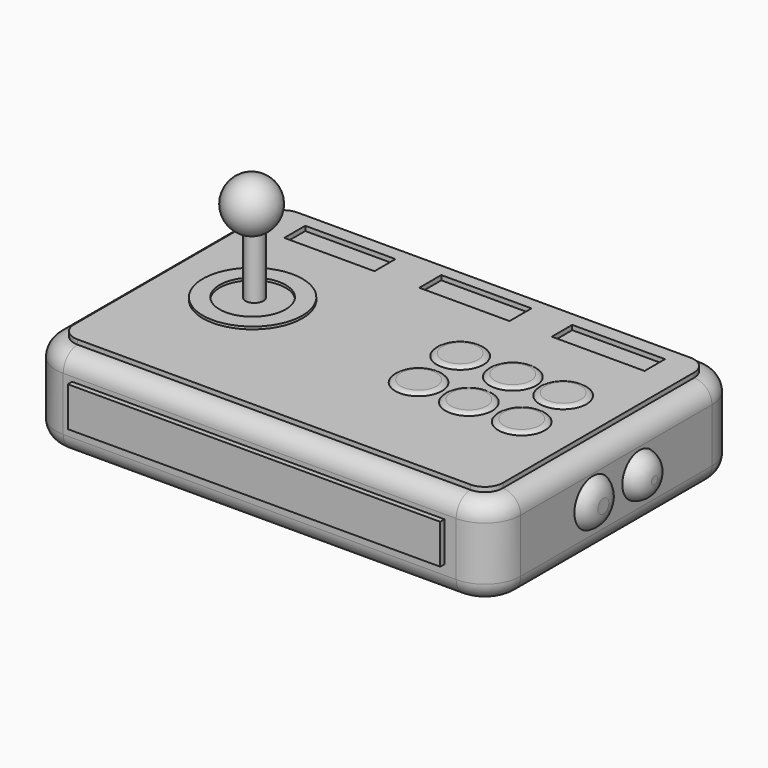
from build123d import *

# Parameters (mm, degrees)
F0_W      = 129.659101367
F0_H      = 86.704544723
F1_DEPTH  = 25
F2_R      = 10
F3_R      = 5
F4_R      = 7
F5_DEPTH  = 2
F4_R_2    = 13.8932950385
F4_R_3    = 9.2347369707
F6_R      = 1.99999
F6_2_R    = 1.99999
F6_3_R    = 1.99999
F6_4_R    = 1.99999
F6_5_R    = 1.99999
F6_6_R    = 1.99999
F7_R      = 2.4900088952
F8_DEPTH  = 18.6
F11_R     = 6.4600643812
F12_DEPTH = 2.9
F14_R     = 5.9996954232
F15_DEPTH = 4.2
F17_W     = 25.178572163
F17_H     = 7.3214266449
F17_H_2   = 7.6785702258
F17_W_2   = 25.8928574622
F17_H_3   = 7.1428548545
F18_DEPTH = 1.3
F19_W     = 22.39266783
F19_H     = 8.6377086118
F19_W_2   = 7.3178783059
F19_H_2   = 7.7066114172
F19_W_3   = 6.5572820604
F19_H_3   = 3.4711612388
F20_DEPTH = 0.7
F21_W     = 103.9311476052
F21_H     = 11.0396803357
F22_DEPTH = 1.5


# Not quite as in the source:
# - a fillet or chamfer that OpenCascade refuses, or shapes differently, is made with other operations: its cross-section is extruded or revolved along the edge and cut away or added
# - a fillet or chamfer is up to 0.001 mm smaller than in the source, because OpenCascade refuses the exact size


with BuildPart() as f1:
    # F0 (on Top) → F1 (new body)
    with BuildSketch(Plane.XY):
        Rectangle(F0_W, F0_H)
    extrude(amount=F1_DEPTH)

    # F2
    f2_edges = [f1.edges().sort_by_distance(p)[0] for p in [
        (-64.829551, -43.352272, 12.5),
        (-64.829551, 43.352272, 12.5),
        (64.829551, -43.352272, 12.5),
        (64.829551, 43.352272, 12.5),
    ]]
    fillet(f2_edges, radius=F2_R)

    # F3
    f3_edges = [f1.edges().sort_by_distance(p)[0] for p in [
        (0, -43.352272, 25),
        (-61.900618, -40.42334, 25),
        (61.900618, -40.42334, 25),
        (-64.829551, 0, 25),
        (64.829551, 0, 25),
        (-61.900618, 40.42334, 25),
        (61.900618, 40.42334, 25),
        (0, 43.352272, 25),
        (0, -43.352272, 0),
        (-61.900618, -40.42334, 0),
        (61.900618, -40.42334, 0),
        (-64.829551, 0, 0),
        (64.829551, 0, 0),
        (-61.900618, 40.42334, 0),
        (61.900618, 40.42334, 0),
        (0, 43.352272, 0),
    ]]
    fillet(f3_edges, radius=F3_R)

    # F7 (on face) → F8 (join)
    with BuildSketch(Plane.XY.offset(25)):
        with Locations((-37.0331034064, 1.0948430281)):
            Circle(F7_R)
    extrude(amount=F8_DEPTH)

    # F9 (on Front) → F10 (revolve)
    with BuildSketch(Plane.XZ):
        with BuildLine():
            Line((-36.9412265718, 49.8054660857), (-36.9412265718, 42.7249787817))
            ThreePointArc((-36.9412265718, 42.7249787817), (-29.8607392679, 49.8054660857), (-36.9412265718, 56.8859533896))
            Line((-36.9412265718, 56.8859533896), (-36.9412265718, 49.8054660857))
        make_face()
    revolve(axis=Axis((-36.9412265718, 0, 53.3457097376), (0, 0, 1)))

    # F11 (on face) → F12 (join)
    with BuildSketch(Plane.YZ.offset(64.8295506835)):
        with Locations((-8.1567466259, 12.9409944639)):
            Circle(F11_R)
    extrude(amount=F12_DEPTH)

    # F13: fillet of radius 5 on 1 edges, made by hand

    # F13_s1 → F13_t2 (revolve, cut)
    with BuildSketch(Plane.XY.offset(12.9409944639)):
        with BuildLine():
            ThreePointArc((64.8295506835, -1.6966822447), (66.9426255701, -3.5417203629), (67.7295506835, -6.2343027665))
            Line((67.7295506835, -6.2343027665), (67.7295506835, -1.6966822447))
            Line((67.7295506835, -1.6966822447), (64.8295506835, -1.6966822447))
        make_face()
    revolve(axis=Axis((67.7295506835, -8.1567466259, 12.9409944639), (1, 0, 0)), mode=Mode.SUBTRACT)

    # F14 (on face) → F15 (join)
    with BuildSketch(Plane.YZ.offset(64.8295506835)):
        with Locations((8.1003680825, 13.1118111312)):
            Circle(F14_R)
    extrude(amount=F15_DEPTH)

    # F16: fillet of radius 5 on 1 edges, made by hand

    # F16_s1 → F16_t2 (revolve, cut)
    with BuildSketch(Plane.XY.offset(13.1118111312)):
        with BuildLine():
            ThreePointArc((64.8295506835, 14.1000635057), (67.8374372364, 12.4048487832), (69.0295506835, 9.164478434))
            Line((69.0295506835, 9.164478434), (69.0295506835, 14.1000635057))
            Line((69.0295506835, 14.1000635057), (64.8295506835, 14.1000635057))
        make_face()
    revolve(axis=Axis((69.0295506835, 8.1003680825, 13.1118111312), (1, 0, 0)), mode=Mode.SUBTRACT)

    # F19 (on face) → F20 (join)
    with BuildSketch(Plane(origin=(0, 43.3522723615, 0), x_dir=(-1, 0, 0), z_dir=(0, 1, 0))):
        with Locations((39.3955782056, 12.2623662464)):
            Rectangle(F19_W, F19_H)
        with Locations((-48.9754192531, 11.7968176492)):
            Rectangle(F19_W_2, F19_H_2)
        with Locations((-36.6080533713, 10.0174429826)):
            Rectangle(F19_W_3, F19_H_3)
    extrude(amount=F20_DEPTH)

    # F21 (on face) → F22 (join)
    with BuildSketch(Plane.XZ.offset(43.3522723615)):
        with Locations((-0.3925319761, 13.2212552708)):
            Rectangle(F21_W, F21_H)
    extrude(amount=F22_DEPTH)


with BuildPart() as f5:
    # F4 (on face) → F5 (new body)
    with BuildSketch(Plane.XY.offset(25)):
        with Locations((15.1755077144, 7.6012640881)):
            Circle(F4_R)
    extrude(amount=F5_DEPTH)

    # F6 (radius 2 in the source; OpenCascade refuses exactly that, so slightly less here)
    f6_edges = [f5.edges().sort_by_distance(p)[0] for p in [
        (8.175508, 7.601264, 27),
    ]]
    fillet(f6_edges, radius=F6_R)


with BuildPart() as f5b:
    # F4 (on face) → F5, piece 2 (new body)
    with BuildSketch(Plane.XY.offset(25)):
        with Locations((30.2891464283, 7.0709597009)):
            Circle(F4_R)
    extrude(amount=F5_DEPTH)

    # F6#2 (radius 2 in the source; OpenCascade refuses exactly that, so slightly less here)
    f6_2_edges = [f5b.edges().sort_by_distance(p)[0] for p in [
        (23.289146, 7.07096, 27),
    ]]
    fillet(f6_2_edges, radius=F6_2_R)


with BuildPart() as f5c:
    # F4 (on face) → F5, piece 3 (new body)
    with BuildSketch(Plane.XY.offset(25)):
        with Locations((44.3421745052, 7.0709597009)):
            Circle(F4_R)
    extrude(amount=F5_DEPTH)

    # F6#3 (radius 2 in the source; OpenCascade refuses exactly that, so slightly less here)
    f6_3_edges = [f5c.edges().sort_by_distance(p)[0] for p in [
        (37.342175, 7.07096, 27),
    ]]
    fillet(f6_3_edges, radius=F6_3_R)


with BuildPart() as f5d:
    # F4 (on face) → F5, piece 4 (new body)
    with BuildSketch(Plane.XY.offset(25)):
        with Locations((15.8871207386, -7.7842059545)):
            Circle(F4_R)
    extrude(amount=F5_DEPTH)

    # F6#4 (radius 2 in the source; OpenCascade refuses exactly that, so slightly less here)
    f6_4_edges = [f5d.edges().sort_by_distance(p)[0] for p in [
        (8.887121, -7.784206, 27),
    ]]
    fillet(f6_4_edges, radius=F6_4_R)


with BuildPart() as f5e:
    # F4 (on face) → F5, piece 5 (new body)
    with BuildSketch(Plane.XY.offset(25)):
        with Locations((30.2548073232, -8.2246502861)):
            Circle(F4_R)
    extrude(amount=F5_DEPTH)

    # F6#5 (radius 2 in the source; OpenCascade refuses exactly that, so slightly less here)
    f6_5_edges = [f5e.edges().sort_by_distance(p)[0] for p in [
        (23.254807, -8.22465, 27),
    ]]
    fillet(f6_5_edges, radius=F6_5_R)


with BuildPart() as f5f:
    # F4 (on face) → F5, piece 6 (new body)
    with BuildSketch(Plane.XY.offset(25)):
        with Locations((45.0025238097, -8.2246502861)):
            Circle(F4_R)
    extrude(amount=F5_DEPTH)

    # F6#6 (radius 2 in the source; OpenCascade refuses exactly that, so slightly less here)
    f6_6_edges = [f5f.edges().sort_by_distance(p)[0] for p in [
        (38.002524, -8.22465, 27),
    ]]
    fillet(f6_6_edges, radius=F6_6_R)


with BuildPart() as f5g:
    # F4 (on face) → F5, piece 7 (new body)
    with BuildSketch(Plane.XY.offset(25)):
        with Locations((-36.6643890738, 0)):
            Circle(F4_R_2)
        with Locations((-36.6643890738, 0)):
            Circle(F4_R_3, mode=Mode.SUBTRACT)
    extrude(amount=F5_DEPTH)


with BuildPart() as f18:
    # F17 (on face) → F18 (new body)
    with BuildSketch(Plane.XY.offset(25)):
        with BuildLine():
            ThreePointArc((-54.8295506835, 38.3522723615), (-58.3650845894, 36.8878062674), (-59.8295506835, 33.3522723615))
            Line((-59.8295506835, 33.3522723615), (-59.8295506835, -33.3522723615))
            ThreePointArc((-59.8295506835, -33.3522723615), (-58.3650845894, -36.8878062674), (-54.8295506835, -38.3522723615))
            Line((-54.8295506835, -38.3522723615), (54.8295506835, -38.3522723615))
            ThreePointArc((54.8295506835, -38.3522723615), (58.3650845894, -36.8878062674), (59.8295506835, -33.3522723615))
            Line((59.8295506835, -33.3522723615), (59.8295506835, 33.3522723615))
            ThreePointArc((59.8295506835, 33.3522723615), (58.3650845894, 36.8878062674), (54.8295506835, 38.3522723615))
            Line((54.8295506835, 38.3522723615), (-54.8295506835, 38.3522723615))
        make_face()
        with Locations((-37.002039142, 30.865653418)):
            Rectangle(F17_W, F17_H, mode=Mode.SUBTRACT)
        with Locations((0.6765332073, 31.0442252085)):
            Rectangle(F17_W, F17_H_2, mode=Mode.SUBTRACT)
        with Locations((37.997962907, 30.7763675228)):
            Rectangle(F17_W_2, F17_H_3, mode=Mode.SUBTRACT)
    extrude(amount=F18_DEPTH)


solid = Compound([f1.part, f5.part, f5b.part, f5c.part, f5d.part, f5e.part, f5f.part, f5g.part, f18.part])
